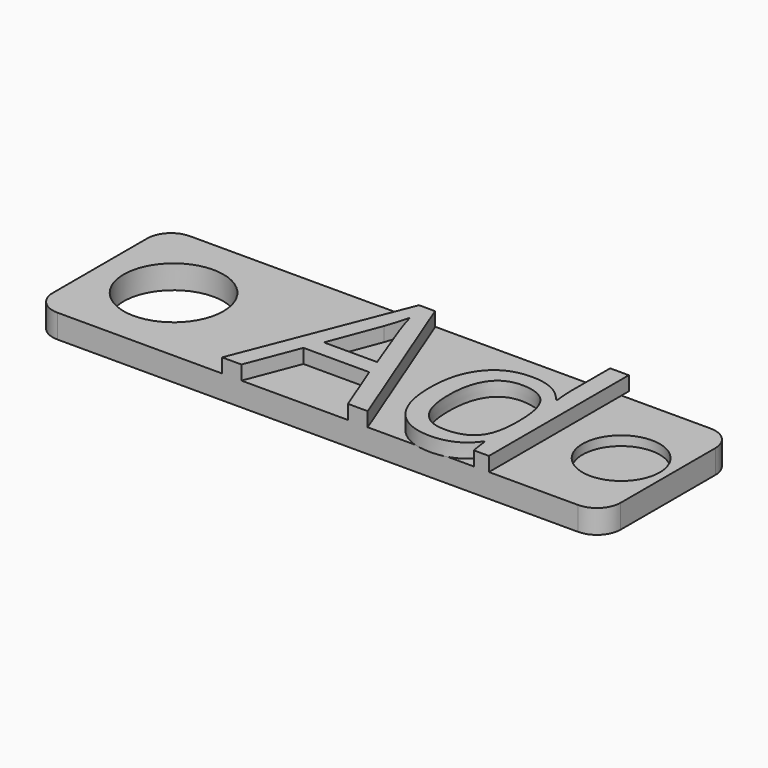
from build123d import *

# Parameters (mm, degrees)
F0_W         = 120
F0_H         = 35
F0_R         = 10.538
F1_DEPTH     = 5
F2_R         = 5
F3_TEXT_SIZE = 48.6111111111
F5_DEPTH     = 3
F4_R         = 8.1607546854
F6_DEPTH     = 2


# Not quite as in the source:
# - Text() gives the source's letters only with a copy of the font that has no kerning and outlines rounded to 1/6400 em; it was checked with that copy


with BuildPart() as f1:
    # F0 (on Top) → F1 (new body)
    with BuildSketch(Plane.XY):
        Rectangle(F0_W, F0_H)
        with Locations((-44.462, 0)):
            Circle(F0_R, mode=Mode.SUBTRACT)
    extrude(amount=F1_DEPTH)

    # F2
    f2_edges = [f1.edges().sort_by_distance(p)[0] for p in [
        (-60, -17.5, 2.5),
        (60, -17.5, 2.5),
        (60, 17.5, 2.5),
        (-60, 17.5, 2.5),
    ]]
    fillet(f2_edges, radius=F2_R)

    # F3 (on face) → F5 (join)
    with BuildSketch(Plane.XY.offset(5)):
        with Locations((-20.203622058, -17.5)):
            Text('Ad', F3_TEXT_SIZE, font='Open Sans', text_align=(TextAlign.LEFT, TextAlign.BOTTOM))
    extrude(amount=F5_DEPTH)

    # F4 (on face) → F6 (cut)
    with BuildSketch(Plane.XY.offset(5)):
        with Locations((50.1018986106, 0)):
            Circle(F4_R)
    extrude(amount=-F6_DEPTH, mode=Mode.SUBTRACT)


solid = f1.part
